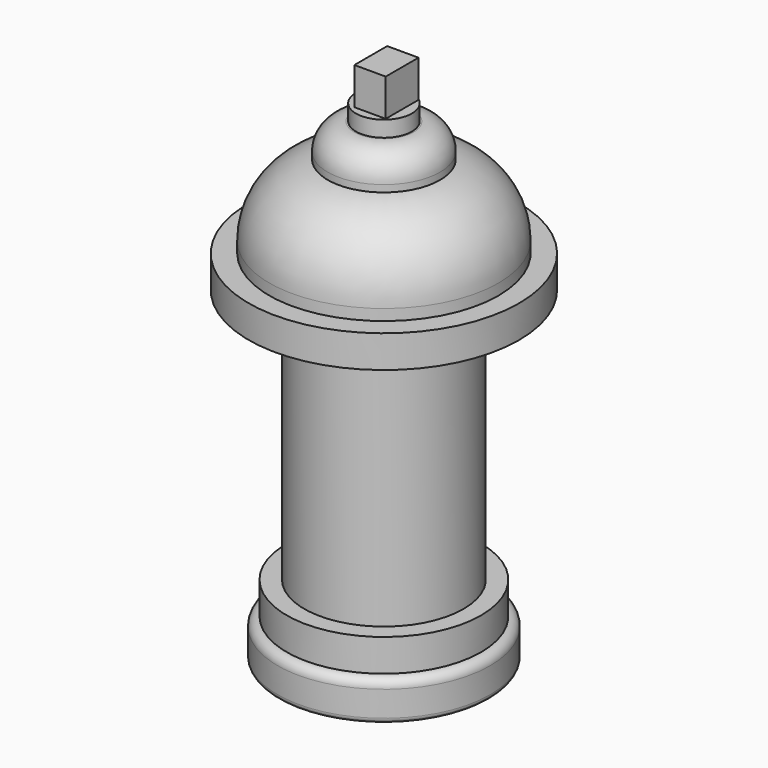
from build123d import *

# Parameters (mm, degrees)
F0_R        = 50.8095284436
F1_DEPTH    = 19.05
F2_R        = 4.318
F3_R        = 2.54
F5_R        = 38.1
F6_DEPTH    = 137.414
F8_R        = 64.7161809078
F1_FACE_R   = 46.4915284436
F1_FACE_R_2 = 38.1
F9_DEPTH    = 15.494
F11_R       = 54.8295431731
F12_DEPTH   = 39.624
F13_R       = 34.3397737112
F15_R       = 26.8787144504
F16_DEPTH   = 16.002
F17_R       = 12.7
F19_R       = 13.3764834425
F20_DEPTH   = 7.62
F22_W       = 15.0005891919
F22_H       = 19.6202434599
F23_DEPTH   = 17.78


with BuildPart() as f1:
    # F0 (on Top) → F1 (new body)
    with BuildSketch(Plane.XY):
        Circle(F0_R)
    extrude(amount=F1_DEPTH)

    # F2
    f2_edges = [f1.edges().sort_by_distance(p)[0] for p in [
        (-50.809528, 0, 19.05),
    ]]
    fillet(f2_edges, radius=F2_R)

    # F3
    f3_edges = [f1.edges().sort_by_distance(p)[0] for p in [
        (-50.809528, 0, 0),
    ]]
    fillet(f3_edges, radius=F3_R)

    # F5 (on offset) → F6 (join)
    with BuildSketch(Plane.XY.offset(19.05)):
        Circle(F5_R)
    extrude(amount=F6_DEPTH)

    # F8 (on offset) + F1_face (on face) → F9 (join)
    with BuildSketch(Plane.XY.offset(156.464)):
        Circle(F8_R)
    with BuildSketch(Plane.XY.offset(19.05)):
        Circle(F1_FACE_R)
        Circle(F1_FACE_R_2, mode=Mode.SUBTRACT)
    extrude(amount=F9_DEPTH)

    # F11 (on offset) → F12 (join)
    with BuildSketch(Plane.XY.offset(171.958)):
        Circle(F11_R)
    extrude(amount=F12_DEPTH)

    # F13
    f13_edges = [f1.edges().sort_by_distance(p)[0] for p in [
        (-54.829543, 0, 211.582),
    ]]
    fillet(f13_edges, radius=F13_R)

    # F15 (on offset) → F16 (join)
    with BuildSketch(Plane.XY.offset(211.582)):
        Circle(F15_R)
    extrude(amount=F16_DEPTH)

    # F17
    f17_edges = [f1.edges().sort_by_distance(p)[0] for p in [
        (-26.878714, 0, 227.584),
    ]]
    fillet(f17_edges, radius=F17_R)

    # F19 (on offset) → F20 (join)
    with BuildSketch(Plane.XY.offset(227.584)):
        Circle(F19_R)
    extrude(amount=F20_DEPTH)

    # F22 (on offset) → F23 (join)
    with BuildSketch(Plane.XY.offset(235.204)):
        with Locations((0.9291712195, 0.3550583497)):
            Rectangle(F22_W, F22_H)
    extrude(amount=F23_DEPTH)


solid = f1.part
